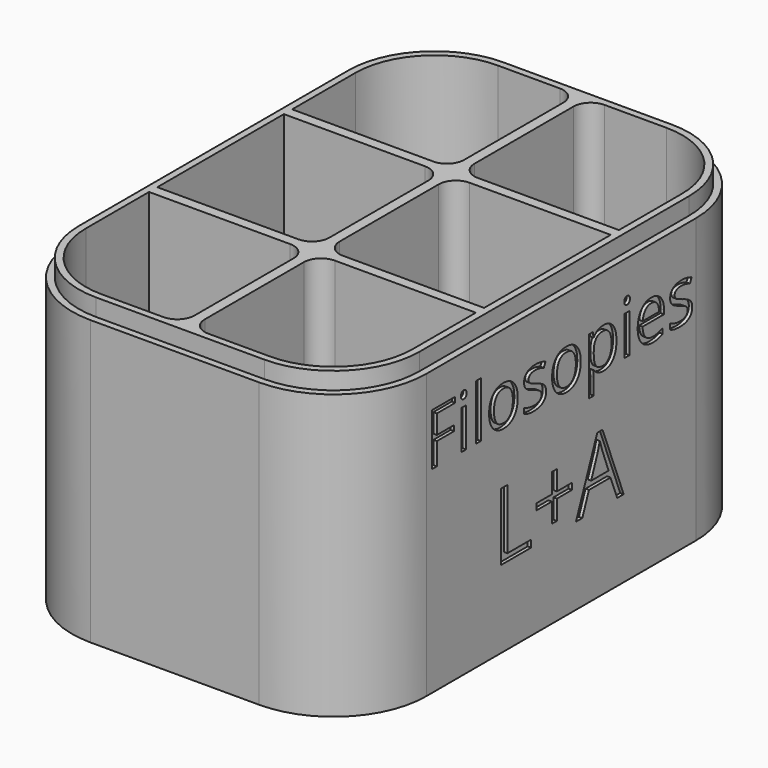
from build123d import *

# Parameters (mm, degrees)
F3_DEPTH        = 2.5
F4_R            = 15
F5_DEPTH        = 5
F6_W            = 46.0000019073
F6_H            = 3
F6_W_2          = 3
F6_H_2          = 46.0000019073
F6_H_3          = 46
F7_DEPTH        = 80
F9_DEPTH        = 5
F10_R           = 5
F11_TEXT_SIZE   = 21.1663066955
F11_TEXT_SIZE_2 = 27.398217718
F12_DEPTH       = 1
F13_TEXT_SIZE   = 21.1663066955
F13_TEXT_SIZE_2 = 27.398217718
F14_DEPTH       = 1


# Not quite as in the source:
# - Text() gives the source's letters only with a copy of the font that has no kerning and outlines rounded to 1/6400 em; it was checked with that copy


with BuildPart() as f3:
    # F2 (on Top) → F3 (new body)
    with BuildSketch(Plane.XY):
        with BuildLine():
            Line((76, 152), (27, 152))
            ThreePointArc((27, 152), (7.908116908, 144.091883092), (0, 125))
            Line((0, 125), (0, 27))
            ThreePointArc((0, 27), (7.908116908, 7.908116908), (27, 0))
            Line((27, 0), (76, 0))
            ThreePointArc((76, 0), (95.091883092, 7.908116908), (103, 27))
            Line((103, 27), (103, 125))
            ThreePointArc((103, 125), (95.091883092, 144.091883092), (76, 152))
        make_face()
    extrude(amount=F3_DEPTH)

    # F4 (on face) → F5 (join)
    with BuildSketch(Plane.XY.offset(2.5)):
        with BuildLine():
            ThreePointArc((103, 125), (95.091883092, 144.091883092), (76, 152))
            Line((76, 152), (27, 152))
            ThreePointArc((27, 152), (7.908116908, 144.091883092), (0, 125))
            Line((0, 125), (0, 27))
            ThreePointArc((0, 27), (7.908116908, 7.908116908), (27, 0))
            Line((27, 0), (76, 0))
            ThreePointArc((76, 0), (95.091883092, 7.908116908), (103, 27))
            Line((103, 27), (103, 125))
        make_face()
        with Locations((27, 27)):
            Circle(F4_R, mode=Mode.SUBTRACT)
        with Locations((76, 27)):
            Circle(F4_R, mode=Mode.SUBTRACT)
        with Locations((27, 76)):
            Circle(F4_R, mode=Mode.SUBTRACT)
        with Locations((27, 125)):
            Circle(F4_R, mode=Mode.SUBTRACT)
        with Locations((76, 76)):
            Circle(F4_R, mode=Mode.SUBTRACT)
        with Locations((76, 125)):
            Circle(F4_R, mode=Mode.SUBTRACT)
    extrude(amount=F5_DEPTH)

    # F6 (on face) → F7 (join)
    with BuildSketch(Plane.XY.offset(7.5)):
        with BuildLine():
            Line((103, 27), (103, 125))
            ThreePointArc((103, 125), (95.091883092, 144.091883092), (76, 152))
            Line((76, 152), (27, 152))
            ThreePointArc((27, 152), (7.908116908, 144.091883092), (0, 125))
            Line((0, 125), (0, 27))
            ThreePointArc((0, 27), (7.908116908, 7.908116908), (27, 0))
            Line((27, 0), (76, 0))
            ThreePointArc((76, 0), (95.091883092, 7.908116908), (103, 27))
        make_face()
        with BuildLine():
            ThreePointArc((3.9999980927, 125), (10.736542684, 141.263457316), (27, 148.0000019073))
            Line((27, 148.0000019073), (50, 148.0000019073))
            Line((50, 148.0000019073), (53, 148.0000019073))
            Line((53, 148.0000019073), (76, 148.0000019073))
            ThreePointArc((76, 148.0000019073), (92.263457316, 141.263457316), (99.0000019073, 125))
            Line((99.0000019073, 125), (99.0000019073, 102))
            Line((99.0000019073, 102), (99.0000019073, 99))
            Line((99.0000019073, 99), (99.0000019073, 53))
            Line((99.0000019073, 53), (99.0000019073, 50))
            Line((99.0000019073, 50), (99.0000019073, 27))
            ThreePointArc((99.0000019073, 27), (92.263457316, 10.736542684), (76, 3.9999980927))
            Line((76, 3.9999980927), (53, 3.9999980927))
            Line((53, 3.9999980927), (50, 3.9999980927))
            Line((50, 3.9999980927), (27, 3.9999980927))
            ThreePointArc((27, 3.9999980927), (10.736542684, 10.736542684), (3.9999980927, 27))
            Line((3.9999980927, 27), (3.9999980927, 50))
            Line((3.9999980927, 50), (3.9999980927, 53))
            Line((3.9999980927, 53), (3.9999980927, 99))
            Line((3.9999980927, 99), (3.9999980927, 102))
            Line((3.9999980927, 102), (3.9999980927, 125))
        make_face(mode=Mode.SUBTRACT)
        with Locations((26.9999990463, 100.5)):
            Rectangle(F6_W, F6_H)
        with Locations((51.5, 100.5)):
            Rectangle(F6_W_2, F6_H)
        with Locations((76.0000009537, 100.5)):
            Rectangle(F6_W, F6_H)
        with Locations((26.9999990463, 51.5)):
            Rectangle(F6_W, F6_H)
        with Locations((51.5, 51.5)):
            Rectangle(F6_W_2, F6_H)
        with Locations((76.0000009537, 51.5)):
            Rectangle(F6_W, F6_H)
        with Locations((51.5, 125.0000009537)):
            Rectangle(F6_W_2, F6_H_2)
        with Locations((51.5, 76)):
            Rectangle(F6_W_2, F6_H_3)
        with Locations((51.5, 26.9999990463)):
            Rectangle(F6_W_2, F6_H_2)
    extrude(amount=F7_DEPTH)

    # F8 (on face) → F9 (cut)
    with BuildSketch(Plane.XY.offset(87.5)):
        with BuildLine():
            Line((27, 0), (76, 0))
            ThreePointArc((76, 0), (95.091883092, 7.908116908), (103, 27))
            Line((103, 27), (103, 125))
            ThreePointArc((103, 125), (95.091883092, 144.091883092), (76, 152))
            Line((76, 152), (27, 152))
            ThreePointArc((27, 152), (7.908116908, 144.091883092), (0, 125))
            Line((0, 125), (0, 27))
            ThreePointArc((0, 27), (7.908116908, 7.908116908), (27, 0))
        make_face()
        with BuildLine():
            ThreePointArc((2, 125), (9.3223304703, 142.6776695297), (27, 150))
            Line((27, 150), (76, 150))
            ThreePointArc((76, 150), (93.6776695297, 142.6776695297), (101, 125))
            Line((101, 125), (101, 27))
            ThreePointArc((101, 27), (93.6776695297, 9.3223304703), (76, 2))
            Line((76, 2), (27, 2))
            ThreePointArc((27, 2), (9.3223304703, 9.3223304703), (2, 27))
            Line((2, 27), (2, 125))
        make_face(mode=Mode.SUBTRACT)
    extrude(amount=-F9_DEPTH, mode=Mode.SUBTRACT)

    # F10
    f10_edges = [f3.edges().sort_by_distance(p)[0] for p in [
        (53, 50, 47.5),
        (50, 50, 47.5),
        (53, 53, 47.5),
        (50, 53, 47.5),
        (50, 102, 47.5),
        (53, 102, 47.5),
        (53, 99, 47.5),
        (50, 99, 47.5),
        (50, 148.000002, 47.5),
        (53, 148.000002, 47.5),
        (50, 3.999998, 47.5),
        (53, 3.999998, 47.5),
    ]]
    fillet(f10_edges, radius=F10_R)

    # F11 (on face) → F12 (cut)
    with BuildSketch(Plane.YZ.offset(103)):
        with Locations((27, 57.2602591793)):
            Text('Filosopies', F11_TEXT_SIZE, font='Open Sans', text_align=(TextAlign.LEFT, TextAlign.BOTTOM))
        with Locations((51.5, 22.5335424223)):
            Text('L+A', F11_TEXT_SIZE_2, font='Open Sans', text_align=(TextAlign.LEFT, TextAlign.BOTTOM))
    extrude(amount=-F12_DEPTH, mode=Mode.SUBTRACT)

    # F13 (on face) → F14 (cut)
    with BuildSketch(Plane(origin=(0, 0, 0), x_dir=(0, -1, 0), z_dir=(-1, 0, 0))):
        with Locations((-125, 57.2602591793)):
            Text('Filosopies', F13_TEXT_SIZE, font='Open Sans', text_align=(TextAlign.LEFT, TextAlign.BOTTOM))
        with Locations((-100.5, 22.5335424223)):
            Text('L+A', F13_TEXT_SIZE_2, font='Open Sans', text_align=(TextAlign.LEFT, TextAlign.BOTTOM))
    extrude(amount=-F14_DEPTH, mode=Mode.SUBTRACT)


solid = f3.part
